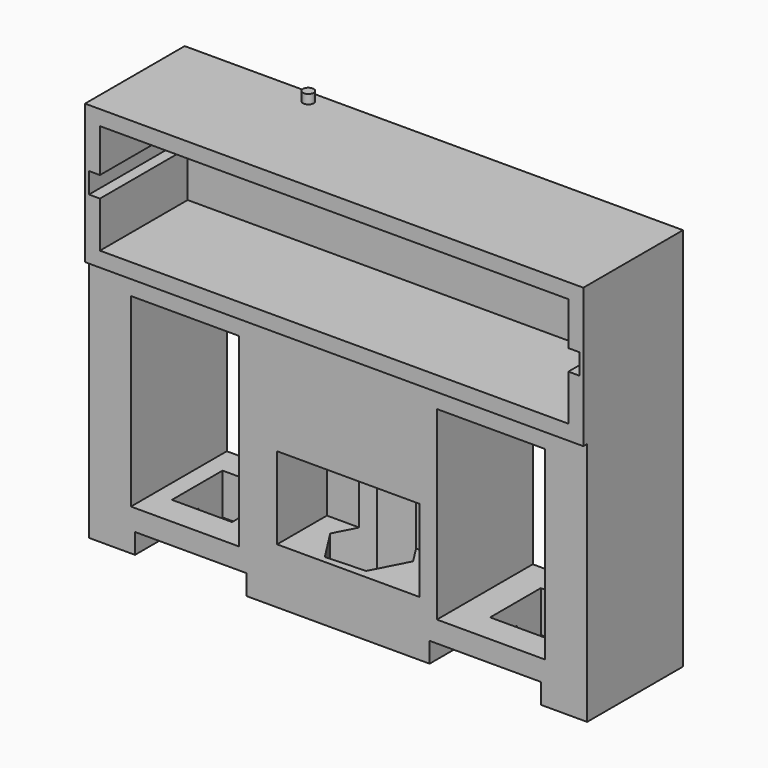
from build123d import *

# Parameters (mm, degrees)
F0_W           = 200
F0_H           = 56
F1_DEPTH       = 50
F2_T           = -6
F3_W           = 149.0980237722
F3_H           = 8.3
F4_DEPTH       = 98.5
F4_DEPTH_BACK  = 98.4
F5_R           = 2.1479446761
F6_DEPTH       = 3.7
F7_W           = 200
F7_H           = 48.0854995549
F8_DEPTH       = 98.2
F9_W           = 44.6983203292
F9_H           = 8.100832057
F10_DEPTH      = 25
F11_W          = 43.396525085
F11_H          = 74.3940398097
F12_DEPTH      = 55.1
F12_DEPTH_BACK = 75
F13_W          = 24.1317078471
F13_H          = 25.4259835929
F14_DEPTH      = 29.4
F16_DEPTH      = 50.3
F17_W          = 57.2261828929
F17_H          = 32.9050645232
F18_DEPTH      = 25


# Not quite as in the source:
# - a pattern or mirror of a feature is missing from the dataset's text; its kind, count and spacing are read off the source's solid


with BuildPart() as f1:
    # F0 (on Front) → F1 (new body)
    with BuildSketch(Plane.XZ):
        Rectangle(F0_W, F0_H)
    extrude(amount=F1_DEPTH)

    # F2
    f2_openings = [f1.faces().sort_by_distance(p)[0] for p in [
        (0, -50, 0),
    ]]
    offset(amount=F2_T, openings=f2_openings)

    # F3 (on Right) → F4 (cut, two sides)
    with BuildSketch(Plane.YZ) as f4_sk:
        with Locations((-82.4490264058, 0.55)):
            Rectangle(F3_W, F3_H)
    extrude(amount=F4_DEPTH, mode=Mode.SUBTRACT)
    extrude(f4_sk.sketch, amount=-F4_DEPTH_BACK, mode=Mode.SUBTRACT)

    # F5 (on face) → F6 (join)
    with BuildSketch(Plane.XY.offset(28)):
        with Locations((-46.3078469038, -5.0663095899)):
            Circle(F5_R)
    extrude(amount=F6_DEPTH)

    # F7 (on face) → F8 (join)
    with BuildSketch(Plane(origin=(0, 0, -28), x_dir=(1, 0, 0), z_dir=(0, 0, -1))):
        with Locations((0, 24.0427497774)):
            Rectangle(F7_W, F7_H)
    extrude(amount=F8_DEPTH)

    # F9 (on face) → F10 (cut)
    with BuildSketch(Plane.XZ.offset(48.0854995549)):
        with Locations((-59.1169446707, -122.1495839715)):
            Rectangle(F9_W, F9_H)
    f10 = extrude(amount=-F10_DEPTH, mode=Mode.SUBTRACT)

    # F10_copies: F10 across plane
    add(f10.mirror(Plane(origin=(0, 0, 0), x_dir=(0, 0, 1), z_dir=(1, 0, 0))), mode=Mode.SUBTRACT)

    # F11 (on Front) → F12 (cut, two sides)
    with BuildSketch(Plane.XZ) as f12_sk:
        with Locations((-61.3989308476, -72.4539384246)):
            Rectangle(F11_W, F11_H)
    f12 = extrude(amount=-F12_DEPTH, mode=Mode.SUBTRACT) + extrude(f12_sk.sketch, amount=F12_DEPTH_BACK, mode=Mode.SUBTRACT)

    # F12_copies: F12 across plane
    add(f12.mirror(Plane(origin=(0, 0, 0), x_dir=(0, 0, 1), z_dir=(1, 0, 0))), mode=Mode.SUBTRACT)

    # F13 (on face) → F14 (cut)
    with BuildSketch(Plane.XY.offset(-109.6509583294)):
        with Locations((-63.8535097241, -23.7910989672)):
            Rectangle(F13_W, F13_H)
    f14 = extrude(amount=-F14_DEPTH, mode=Mode.SUBTRACT)

    # F14_copies: F14 across plane
    add(f14.mirror(Plane(origin=(0, 0, 0), x_dir=(0, 0, 1), z_dir=(1, 0, 0))), mode=Mode.SUBTRACT)

    # F15 (on face) → F16 (cut)
    with BuildSketch(Plane(origin=(0, 0, -126.2), x_dir=(1, 0, 0), z_dir=(0, 0, -1))):
        Polygon((16.0494638515, 30.4643716825), (8.6599005478, 44.7303298699), (-7.3895633037, 45.4637594198), (-16.0494638515, 31.9312307822), (-8.6599005478, 17.6652725948), (7.3895633037, 16.9318430449), align=None)
    extrude(amount=-F16_DEPTH, mode=Mode.SUBTRACT)

    # F17 (on face) → F18 (cut)
    with BuildSketch(Plane.XZ.offset(48.0854995549)):
        with Locations((4.1727414355, -87.4758176506)):
            Rectangle(F17_W, F17_H)
    extrude(amount=-F18_DEPTH, mode=Mode.SUBTRACT)


solid = f1.part
